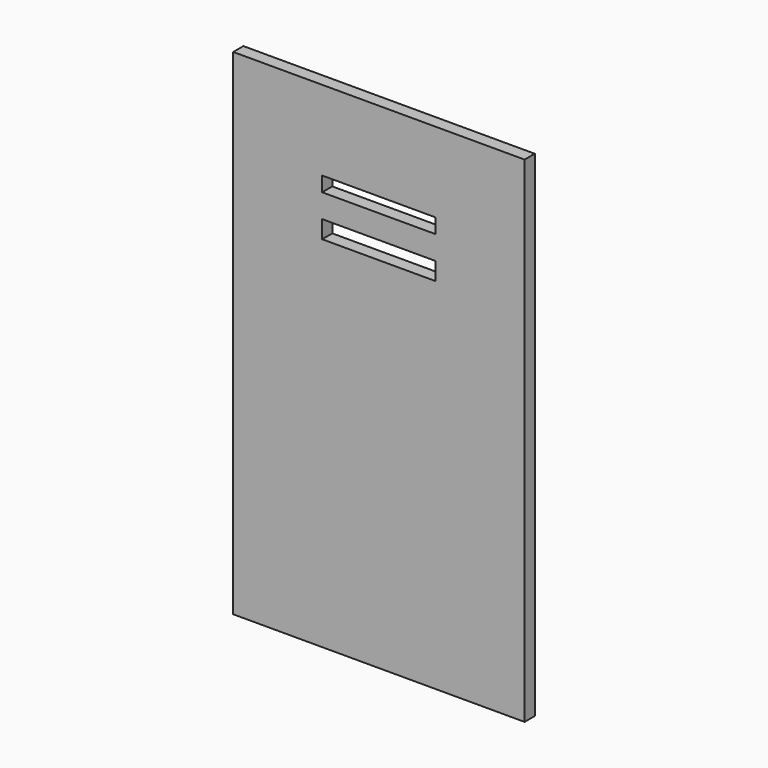
from build123d import *

# Parameters (mm, degrees)
F0_W           = 290.9753695428
F0_H           = 494.4017827511
F0_W_2         = 113.365188241
F0_H_2         = 17.700329423
F0_H_3         = 14.7502720356
F1_DEPTH       = 12.7
F2_TEXT_SIZE   = 53.2648422652
F3_DEPTH       = 7.62
F4_R           = 38.0898351173
F5_DEPTH       = 10.16
F6_R           = 27.9181972255
F7_DEPTH       = 7.62
F8_TEXT_SIZE   = 10.4799711456
F8_TEXT_SIZE_2 = 10.4799704988
F8_TEXT_SIZE_3 = 9.1277140503
F8_TEXT_SIZE_4 = 10.4340110233
F9_DEPTH       = 2.54


# Not quite as in the source:
# - Text() gives the source's letters only with a copy of the font that has no kerning and outlines rounded to 1/6400 em; it was checked with that copy


with BuildPart() as f1:
    # F0 (on Front) → F1 (new body)
    with BuildSketch(Plane.XZ):
        Rectangle(F0_W, F0_H)
        with Locations((0, 120.2722936869)):
            Rectangle(F0_W_2, F0_H_2, mode=Mode.SUBTRACT)
        with Locations((0, 160.0980013609)):
            Rectangle(F0_W_2, F0_H_3, mode=Mode.SUBTRACT)
    extrude(amount=F1_DEPTH)

    # F2 (on face) → F3 (join)
    with BuildSketch(Plane(origin=(0, 0, 0), x_dir=(-1, 0, 0), z_dir=(0, 1, 0))):
        with Locations((-56.6825941205, 37.6708060503)):
            Text('1116', F2_TEXT_SIZE, font='Open Sans', text_align=(TextAlign.LEFT, TextAlign.BOTTOM))
    extrude(amount=F3_DEPTH)

    # F4 (on face) → F5 (join)
    with BuildSketch(Plane(origin=(0, 0, 0), x_dir=(-1, 0, 0), z_dir=(0, 1, 0))):
        Circle(F4_R)
    extrude(amount=F5_DEPTH)

    # F6 (on face) → F7 (join)
    with BuildSketch(Plane(origin=(0, 10.16, 0), x_dir=(-1, 0, 0), z_dir=(0, 1, 0))):
        Circle(F6_R)
    extrude(amount=F7_DEPTH)

    # F8 (on face) → F9 (join)
    with BuildSketch(Plane(origin=(0, 17.78, 0), x_dir=(-1, 0, 0), z_dir=(0, 1, 0))):
        with Locations((-3.8416229654, 17.0053131878)):
            Text('1', F8_TEXT_SIZE, font='Open Sans', text_align=(TextAlign.LEFT, TextAlign.BOTTOM))
        with Locations((13.1599027663, 0.1486269757)):
            Text('30', F8_TEXT_SIZE_2, font='Open Sans', text_align=(TextAlign.LEFT, TextAlign.BOTTOM))
        with Locations((-2.381188795, -24.8604789376)):
            Text('60', F8_TEXT_SIZE_3, font='Open Sans', text_align=(TextAlign.LEFT, TextAlign.BOTTOM))
        with Locations((-22.8272732347, 0)):
            Text('90', F8_TEXT_SIZE_4, font='Open Sans', text_align=(TextAlign.LEFT, TextAlign.BOTTOM))
    extrude(amount=F9_DEPTH)


solid = f1.part
